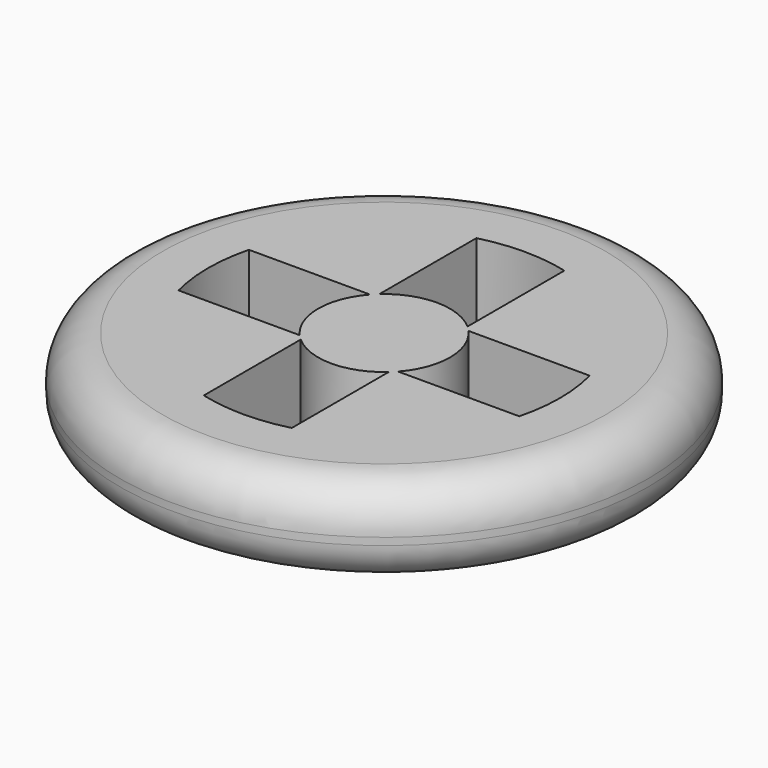
from build123d import *

# Parameters (mm, degrees)
F0_R     = 76.2
F1_DEPTH = 12.7
F2_R     = 12.2642048969
F3_R     = 11.0377844072


# Not quite as in the source:
# - ends of sketch curves that miss each other by under 0.0002 mm in the source are joined
# - a feature names something its author has since deleted; it is built from what else it names


with BuildPart() as f1:
    # F0 (on Top) → F1 (new body, symmetric)
    with BuildSketch(Plane.XY):
        Circle(F0_R)
        with BuildLine():
            ThreePointArc((49.1868885365, 12.6999998465), (50.3951085804, 6.4010179795), (50.8, 0))
            ThreePointArc((50.8, 0), (50.3951085804, -6.4010179795), (49.1868885365, -12.6999998465))
            ThreePointArc((49.1868885365, -12.6999998465), (35.9210245403, -35.9210244282), (12.7, -49.1868884968))
            ThreePointArc((12.7, -49.1868884968), (6.4010180581, -50.3951085704), (0, -50.8))
            ThreePointArc((0, -50.8), (-6.4010180581, -50.3951085704), (-12.7, -49.1868884968))
            ThreePointArc((-12.7, -49.1868884968), (-35.9210245403, -35.9210244282), (-49.1868885365, -12.6999998465))
            ThreePointArc((-49.1868885365, -12.6999998465), (-50.3951085804, -6.4010179795), (-50.8, 0))
            ThreePointArc((-50.8, 0), (-50.3951085704, 6.4010180581), (-49.1868884968, 12.7))
            ThreePointArc((-49.1868884968, 12.7), (-35.9210244282, 35.9210245403), (-12.6999998465, 49.1868885365))
            ThreePointArc((-12.6999998465, 49.1868885365), (-6.4010179795, 50.3951085804), (0, 50.8))
            ThreePointArc((0, 50.8), (6.4010179795, 50.3951085804), (12.6999998465, 49.1868885365))
            ThreePointArc((12.6999998465, 49.1868885365), (35.9210244843, 35.9210244843), (49.1868885365, 12.6999998465))
        make_face(mode=Mode.SUBTRACT)
        with BuildLine():
            ThreePointArc((12.7, -49.1868884968), (35.9210245403, -35.9210244282), (49.1868885365, -12.6999998465))
            Line((49.1868885365, -12.6999998465), (14.1990317944, -12.6999998465))
            Line((14.1990317944, -12.6999998465), (12.7, -12.6999998465))
            Line((12.7, -12.6999998465), (12.7, -14.1990316571))
            Line((12.7, -14.1990316571), (12.7, -49.1868884968))
        make_face()
        with BuildLine():
            ThreePointArc((-49.1868885365, -12.6999998465), (-35.9210245403, -35.9210244282), (-12.7, -49.1868884968))
            Line((-12.7, -49.1868884968), (-12.7, -14.1990316571))
            Line((-12.7, -14.1990316571), (-12.7, -12.6999998465))
            Line((-12.7, -12.6999998465), (-14.1990317944, -12.6999998465))
            Line((-14.1990317944, -12.6999998465), (-49.1868885365, -12.6999998465))
        make_face()
        with BuildLine():
            Line((-12.6999998465, 14.1990317944), (-12.6999998465, 49.1868885365))
            ThreePointArc((-12.6999998465, 49.1868885365), (-35.9210244282, 35.9210245403), (-49.1868884968, 12.7))
            Line((-49.1868884968, 12.7), (-14.1990316571, 12.7))
            Line((-14.1990316571, 12.7), (-12.6999998465, 12.7))
            Line((-12.6999998465, 12.7), (-12.6999998465, 14.1990317944))
        make_face()
        with BuildLine():
            Line((14.1990317944, 12.6999998465), (49.1868885365, 12.6999998465))
            ThreePointArc((49.1868885365, 12.6999998465), (35.9210244843, 35.9210244843), (12.6999998465, 49.1868885365))
            Line((12.6999998465, 49.1868885365), (12.6999998465, 14.1990317944))
            Line((12.6999998465, 14.1990317944), (12.6999998465, 12.6999998465))
            Line((12.6999998465, 12.6999998465), (14.1990317944, 12.6999998465))
        make_face()
        Polygon((12.7, -12.6999998465), (12.7, 0), (12.6999998465, 12.6999998465), (0, 12.6999998465), (-12.6999998465, 12.7), (-12.7, 0), (-12.7, -12.6999998465), (0, -12.6999998465), align=None)
        with BuildLine():
            Line((-12.7, 0), (-12.6999998465, 12.7))
            Line((-12.6999998465, 12.7), (-14.1990316571, 12.7))
            ThreePointArc((-14.1990316571, 12.7), (-17.7959834382, 6.7974608102), (-19.05, 0))
            Line((-19.05, 0), (-12.7, 0))
        make_face()
        with BuildLine():
            ThreePointArc((14.1990317944, -12.6999998465), (17.795983475, -6.797460714), (19.05, 0))
            Line((19.05, 0), (12.7, 0))
            Line((12.7, 0), (12.7, -12.6999998465))
            Line((12.7, -12.6999998465), (14.1990317944, -12.6999998465))
        make_face()
        with BuildLine():
            Line((12.7, 0), (19.05, 0))
            ThreePointArc((19.05, 0), (17.795983475, 6.797460714), (14.1990317944, 12.6999998465))
            Line((14.1990317944, 12.6999998465), (12.6999998465, 12.6999998465))
            Line((12.6999998465, 12.6999998465), (12.7, 0))
        make_face()
        with BuildLine():
            ThreePointArc((0, -19.05), (6.7974608102, -17.7959834382), (12.7, -14.1990316571))
            Line((12.7, -14.1990316571), (12.7, -12.6999998465))
            Line((12.7, -12.6999998465), (0, -12.6999998465))
            Line((0, -12.6999998465), (0, -19.05))
        make_face()
        with BuildLine():
            ThreePointArc((-12.7, -14.1990316571), (-6.7974608102, -17.7959834382), (0, -19.05))
            Line((0, -19.05), (0, -12.6999998465))
            Line((0, -12.6999998465), (-12.7, -12.6999998465))
            Line((-12.7, -12.6999998465), (-12.7, -14.1990316571))
        make_face()
        with BuildLine():
            Line((-14.1990317944, -12.6999998465), (-12.7, -12.6999998465))
            Line((-12.7, -12.6999998465), (-12.7, 0))
            Line((-12.7, 0), (-19.05, 0))
            ThreePointArc((-19.05, 0), (-17.795983475, -6.797460714), (-14.1990317944, -12.6999998465))
        make_face()
        with BuildLine():
            Line((0, 12.6999998465), (0, 19.05))
            ThreePointArc((0, 19.05), (-6.797460714, 17.795983475), (-12.6999998465, 14.1990317944))
            Line((-12.6999998465, 14.1990317944), (-12.6999998465, 12.7))
            Line((-12.6999998465, 12.7), (0, 12.6999998465))
        make_face()
        with BuildLine():
            Line((12.6999998465, 12.6999998465), (12.6999998465, 14.1990317944))
            ThreePointArc((12.6999998465, 14.1990317944), (6.797460714, 17.795983475), (0, 19.05))
            Line((0, 19.05), (0, 12.6999998465))
            Line((0, 12.6999998465), (12.6999998465, 12.6999998465))
        make_face()
    extrude(amount=F1_DEPTH, both=True)

    # F2
    f2_edges = [f1.edges().sort_by_distance(p)[0] for p in [
        (-76.2, 0, 12.7),
    ]]
    fillet(f2_edges, radius=F2_R)

    # F3
    f3_edges = [f1.edges().sort_by_distance(p)[0] for p in [
        (-76.2, 0, -12.7),
    ]]
    fillet(f3_edges, radius=F3_R)


solid = f1.part
